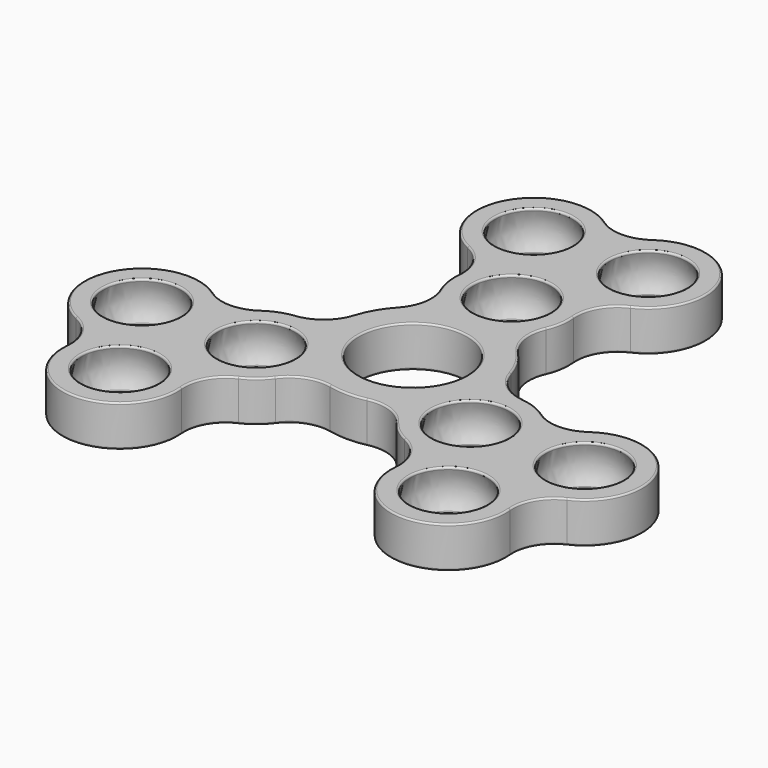
from build123d import *

# Parameters (mm, degrees)
F0_R     = 2.5
F0_R_2   = 6.56
F1_DEPTH = 2.5
F2_DEPTH = 2.5
F22_R    = 0.2


with BuildPart() as f1:
    # F0 (on Top) → F1 (new body)
    with BuildSketch(Plane.XY):
        with BuildLine():
            ThreePointArc((66.8263440398, 12.8050629308), (67.1732713624, 9.9684029043), (65.9098289008, 7.4050629308))
            ThreePointArc((65.9098289008, 7.4050629308), (64.5816959749, 5.6050629308), (63.686916711, 3.5548660774))
            ThreePointArc((63.686916711, 3.5548660774), (62.0987204063, 1.1790228227), (59.4686371001, 0.0611406841))
            ThreePointArc((59.4686371001, 0.0611406841), (57.7608978106, -0.3530293011), (56.2101170716, -1.1794610027))
            ThreePointArc((56.2101170716, -1.1794610027), (53.3233657257, -2.096978098), (50.4366143798, -1.1794610027))
            ThreePointArc((50.4366143798, -1.1794610027), (40.3329846689, -3.3949370692), (43.4661409693, -13.2526751024))
            ThreePointArc((43.4661409693, -13.2526751024), (45.7041097552, -15.2939165547), (46.3528923152, -18.2526751024))
            ThreePointArc((46.3528923152, -18.2526751024), (53.3233657257, -25.8949370692), (60.2938391362, -18.2526751024))
            ThreePointArc((60.2938391362, -18.2526751024), (60.9426216962, -15.2939165547), (63.1805904821, -13.2526751024))
            ThreePointArc((63.1805904821, -13.2526751024), (64.6716916996, -12.3228754376), (65.884243073, -11.0510148224))
            ThreePointArc((65.884243073, -11.0510148224), (68.1673990566, -9.3322369345), (71.019037823, -9.1447402157))
            ThreePointArc((71.019037823, -9.1447402157), (73.2419500127, -9.3949370692), (75.4648622025, -9.1447402157))
            ThreePointArc((75.4648622025, -9.1447402157), (78.3165009689, -9.3322369345), (80.5996569524, -11.0510148224))
            ThreePointArc((80.5996569524, -11.0510148224), (81.8122083259, -12.3228754376), (83.3033095434, -13.2526751024))
            ThreePointArc((83.3033095434, -13.2526751024), (85.5412783293, -15.2939165547), (86.1900608893, -18.2526751024))
            ThreePointArc((86.1900608893, -18.2526751024), (93.1605342998, -25.8949370692), (100.1310077103, -18.2526751024))
            ThreePointArc((100.1310077103, -18.2526751024), (100.7797902702, -15.2939165547), (103.0177590562, -13.2526751024))
            ThreePointArc((103.0177590562, -13.2526751024), (106.1509153566, -3.3949370692), (96.0472856457, -1.1794610027))
            ThreePointArc((96.0472856457, -1.1794610027), (93.1605342998, -2.096978098), (90.2737829538, -1.1794610027))
            ThreePointArc((90.2737829538, -1.1794610027), (88.7230022149, -0.3530293011), (87.0152629254, 0.0611406841))
            ThreePointArc((87.0152629254, 0.0611406841), (84.3851796192, 1.1790228227), (82.7969833144, 3.5548660774))
            ThreePointArc((82.7969833144, 3.5548660774), (81.9022040506, 5.6050629308), (80.5740711247, 7.4050629308))
            ThreePointArc((80.5740711247, 7.4050629308), (79.3106286631, 9.9684029043), (79.6575559857, 12.8050629308))
            ThreePointArc((79.6575559857, 12.8050629308), (80.1527439018, 14.4910935312), (80.2124234232, 16.2473248976))
            ThreePointArc((80.2124234232, 16.2473248976), (80.8612059832, 19.2060834453), (83.0991747692, 21.2473248976))
            ThreePointArc((83.0991747692, 21.2473248976), (86.2323310695, 31.1050629308), (76.1287013587, 33.3205389973))
            ThreePointArc((76.1287013587, 33.3205389973), (73.2419500127, 32.403021902), (70.3551986668, 33.3205389973))
            ThreePointArc((70.3551986668, 33.3205389973), (60.251568956, 31.1050629308), (63.3847252563, 21.2473248976))
            ThreePointArc((63.3847252563, 21.2473248976), (65.6226940423, 19.2060834453), (66.2714766023, 16.2473248976))
            ThreePointArc((66.2714766023, 16.2473248976), (66.3311561237, 14.4910935312), (66.8263440398, 12.8050629308))
        make_face()
        with Locations((53.3233657257, -18.8949370692)):
            Circle(F0_R, mode=Mode.SUBTRACT)
        with Locations((46.3951624954, -6.8949370692)):
            Circle(F0_R, mode=Mode.SUBTRACT)
        with Locations((60.251568956, -6.8949370692)):
            Circle(F0_R, mode=Mode.SUBTRACT)
        with Locations((73.2419500127, 0.6050629308)):
            Circle(F0_R_2, mode=Mode.SUBTRACT)
        with Locations((93.1605342998, -18.8949370692)):
            Circle(F0_R, mode=Mode.SUBTRACT)
        with Locations((86.2323310695, -6.8949370692)):
            Circle(F0_R, mode=Mode.SUBTRACT)
        with Locations((100.0887375301, -6.8949370692)):
            Circle(F0_R, mode=Mode.SUBTRACT)
        with Locations((73.2419500127, 15.6050629308)):
            Circle(F0_R, mode=Mode.SUBTRACT)
        with Locations((66.3137467825, 27.6050629308)):
            Circle(F0_R, mode=Mode.SUBTRACT)
        with Locations((80.170153243, 27.6050629308)):
            Circle(F0_R, mode=Mode.SUBTRACT)
    extrude(amount=F1_DEPTH)

    # F0 (on Top) → F2 (join)
    with BuildSketch(Plane.XY):
        with BuildLine():
            ThreePointArc((66.8263440398, 12.8050629308), (67.1732713624, 9.9684029043), (65.9098289008, 7.4050629308))
            ThreePointArc((65.9098289008, 7.4050629308), (64.5816959749, 5.6050629308), (63.686916711, 3.5548660774))
            ThreePointArc((63.686916711, 3.5548660774), (62.0987204063, 1.1790228227), (59.4686371001, 0.0611406841))
            ThreePointArc((59.4686371001, 0.0611406841), (57.7608978106, -0.3530293011), (56.2101170716, -1.1794610027))
            ThreePointArc((56.2101170716, -1.1794610027), (53.3233657257, -2.096978098), (50.4366143798, -1.1794610027))
            ThreePointArc((50.4366143798, -1.1794610027), (40.3329846689, -3.3949370692), (43.4661409693, -13.2526751024))
            ThreePointArc((43.4661409693, -13.2526751024), (45.7041097552, -15.2939165547), (46.3528923152, -18.2526751024))
            ThreePointArc((46.3528923152, -18.2526751024), (53.3233657257, -25.8949370692), (60.2938391362, -18.2526751024))
            ThreePointArc((60.2938391362, -18.2526751024), (60.9426216962, -15.2939165547), (63.1805904821, -13.2526751024))
            ThreePointArc((63.1805904821, -13.2526751024), (64.6716916996, -12.3228754376), (65.884243073, -11.0510148224))
            ThreePointArc((65.884243073, -11.0510148224), (68.1673990566, -9.3322369345), (71.019037823, -9.1447402157))
            ThreePointArc((71.019037823, -9.1447402157), (73.2419500127, -9.3949370692), (75.4648622025, -9.1447402157))
            ThreePointArc((75.4648622025, -9.1447402157), (78.3165009689, -9.3322369345), (80.5996569524, -11.0510148224))
            ThreePointArc((80.5996569524, -11.0510148224), (81.8122083259, -12.3228754376), (83.3033095434, -13.2526751024))
            ThreePointArc((83.3033095434, -13.2526751024), (85.5412783293, -15.2939165547), (86.1900608893, -18.2526751024))
            ThreePointArc((86.1900608893, -18.2526751024), (93.1605342998, -25.8949370692), (100.1310077103, -18.2526751024))
            ThreePointArc((100.1310077103, -18.2526751024), (100.7797902702, -15.2939165547), (103.0177590562, -13.2526751024))
            ThreePointArc((103.0177590562, -13.2526751024), (106.1509153566, -3.3949370692), (96.0472856457, -1.1794610027))
            ThreePointArc((96.0472856457, -1.1794610027), (93.1605342998, -2.096978098), (90.2737829538, -1.1794610027))
            ThreePointArc((90.2737829538, -1.1794610027), (88.7230022149, -0.3530293011), (87.0152629254, 0.0611406841))
            ThreePointArc((87.0152629254, 0.0611406841), (84.3851796192, 1.1790228227), (82.7969833144, 3.5548660774))
            ThreePointArc((82.7969833144, 3.5548660774), (81.9022040506, 5.6050629308), (80.5740711247, 7.4050629308))
            ThreePointArc((80.5740711247, 7.4050629308), (79.3106286631, 9.9684029043), (79.6575559857, 12.8050629308))
            ThreePointArc((79.6575559857, 12.8050629308), (80.1527439018, 14.4910935312), (80.2124234232, 16.2473248976))
            ThreePointArc((80.2124234232, 16.2473248976), (80.8612059832, 19.2060834453), (83.0991747692, 21.2473248976))
            ThreePointArc((83.0991747692, 21.2473248976), (86.2323310695, 31.1050629308), (76.1287013587, 33.3205389973))
            ThreePointArc((76.1287013587, 33.3205389973), (73.2419500127, 32.403021902), (70.3551986668, 33.3205389973))
            ThreePointArc((70.3551986668, 33.3205389973), (60.251568956, 31.1050629308), (63.3847252563, 21.2473248976))
            ThreePointArc((63.3847252563, 21.2473248976), (65.6226940423, 19.2060834453), (66.2714766023, 16.2473248976))
            ThreePointArc((66.2714766023, 16.2473248976), (66.3311561237, 14.4910935312), (66.8263440398, 12.8050629308))
        make_face()
        with Locations((53.3233657257, -18.8949370692)):
            Circle(F0_R, mode=Mode.SUBTRACT)
        with Locations((46.3951624954, -6.8949370692)):
            Circle(F0_R, mode=Mode.SUBTRACT)
        with Locations((60.251568956, -6.8949370692)):
            Circle(F0_R, mode=Mode.SUBTRACT)
        with Locations((73.2419500127, 0.6050629308)):
            Circle(F0_R_2, mode=Mode.SUBTRACT)
        with Locations((93.1605342998, -18.8949370692)):
            Circle(F0_R, mode=Mode.SUBTRACT)
        with Locations((86.2323310695, -6.8949370692)):
            Circle(F0_R, mode=Mode.SUBTRACT)
        with Locations((100.0887375301, -6.8949370692)):
            Circle(F0_R, mode=Mode.SUBTRACT)
        with Locations((73.2419500127, 15.6050629308)):
            Circle(F0_R, mode=Mode.SUBTRACT)
        with Locations((66.3137467825, 27.6050629308)):
            Circle(F0_R, mode=Mode.SUBTRACT)
        with Locations((80.170153243, 27.6050629308)):
            Circle(F0_R, mode=Mode.SUBTRACT)
    extrude(amount=-F2_DEPTH)


with BuildPart() as f4:
    # F3 (on face) → F4 (revolve)
    with BuildSketch(Plane.XY):
        with BuildLine():
            Line((53.3233657257, -24.1049370692), (53.3233657257, -18.8949370692))
            Line((53.3233657257, -18.8949370692), (53.3233657257, -13.6849370692))
            ThreePointArc((53.3233657257, -13.6849370692), (48.1133657257, -18.8949370692), (53.3233657257, -24.1049370692))
        make_face()
    revolve(axis=Axis((53.3233657257, -16.2899370692, 0), (0, 1, 0)))


with BuildPart() as f7:
    # F6 (on face) → F7 (revolve)
    with BuildSketch(Plane.XY):
        with BuildLine():
            Line((93.1605342998, -24.1049370692), (93.1605342998, -18.8949370692))
            Line((93.1605342998, -18.8949370692), (93.1605342998, -13.6849370692))
            ThreePointArc((93.1605342998, -13.6849370692), (87.9505342998, -18.8949370692), (93.1605342998, -24.1049370692))
        make_face()
    revolve(axis=Axis((93.1605342998, -16.2899370692, 0), (0, 1, 0)))


with BuildPart() as f9:
    # F8 (on face) → F9 (revolve)
    with BuildSketch(Plane.XY):
        with BuildLine():
            Line((86.2323310695, -12.1049370692), (86.2323310695, -6.8949370692))
            Line((86.2323310695, -6.8949370692), (86.2323310695, -1.6849370692))
            ThreePointArc((86.2323310695, -1.6849370692), (81.0223310695, -6.8949370692), (86.2323310695, -12.1049370692))
        make_face()
    revolve(axis=Axis((86.2323310695, -4.2899370692, 0), (0, 1, 0)))


with BuildPart() as f11:
    # F10 (on face) → F11 (revolve)
    with BuildSketch(Plane.XY):
        with BuildLine():
            Line((100.0887375301, -12.1049370692), (100.0887375301, -6.8949370692))
            Line((100.0887375301, -6.8949370692), (100.0887375301, -1.6849370692))
            ThreePointArc((100.0887375301, -1.6849370692), (94.8787375301, -6.8949370692), (100.0887375301, -12.1049370692))
        make_face()
    revolve(axis=Axis((100.0887375301, -9.4999370692, 0), (0, -1, 0)))


with BuildPart() as f13:
    # F12 (on face) → F13 (revolve)
    with BuildSketch(Plane.XY):
        with BuildLine():
            Line((73.2419500127, 10.3950629308), (73.2419500127, 15.6050629308))
            Line((73.2419500127, 15.6050629308), (73.2419500127, 20.8150629308))
            ThreePointArc((73.2419500127, 20.8150629308), (68.0319500127, 15.6050629308), (73.2419500127, 10.3950629308))
        make_face()
    revolve(axis=Axis((73.2419500127, 13.0000629308, 0), (0, -1, 0)))


with BuildPart() as f15:
    # F14 (on face) → F15 (revolve)
    with BuildSketch(Plane.XY):
        with BuildLine():
            Line((66.3137467825, 22.3950629308), (66.3137467825, 27.6050629308))
            Line((66.3137467825, 27.6050629308), (66.3137467825, 32.8150629308))
            ThreePointArc((66.3137467825, 32.8150629308), (61.1037467825, 27.6050629308), (66.3137467825, 22.3950629308))
        make_face()
    revolve(axis=Axis((66.3137467825, 25.0000629308, 0), (0, -1, 0)))


with BuildPart() as f17:
    # F5 (on face) → F17 (revolve)
    with BuildSketch(Plane.XY):
        with BuildLine():
            Line((60.251568956, -12.1049370692), (60.251568956, -6.8949370692))
            Line((60.251568956, -6.8949370692), (60.251568956, -1.6849370692))
            ThreePointArc((60.251568956, -1.6849370692), (55.041568956, -6.8949370692), (60.251568956, -12.1049370692))
        make_face()
    revolve(axis=Axis((60.251568956, -4.2899370692, 0), (0, 1, 0)))


with BuildPart() as f18:
    # F16 (on face) → F18 (revolve)
    with BuildSketch(Plane.XY):
        with BuildLine():
            Line((80.170153243, 22.3950629308), (80.170153243, 27.6050629308))
            Line((80.170153243, 27.6050629308), (80.170153243, 32.8150629308))
            ThreePointArc((80.170153243, 32.8150629308), (74.960153243, 27.6050629308), (80.170153243, 22.3950629308))
        make_face()
    revolve(axis=Axis((80.170153243, 25.0000629308, 0), (0, -1, 0)))


with BuildPart() as f20:
    # F19 (on face) → F20 (revolve)
    with BuildSketch(Plane.XY):
        with BuildLine():
            Line((46.3951624954, -12.1049370692), (46.3951624954, -6.8949370692))
            Line((46.3951624954, -6.8949370692), (46.3951624954, -1.6849370692))
            ThreePointArc((46.3951624954, -1.6849370692), (41.1851624954, -6.8949370692), (46.3951624954, -12.1049370692))
        make_face()
    revolve(axis=Axis((46.3951624954, -9.4999370692, 0), (0, -1, 0)))


with BuildPart() as f1_1:
    add(f1.part)

    # F21: cut F15, F18, F13, F9, F11, F20, F17, F4, F7
    add(f15.part, mode=Mode.SUBTRACT)
    add(f18.part, mode=Mode.SUBTRACT)
    add(f13.part, mode=Mode.SUBTRACT)
    add(f9.part, mode=Mode.SUBTRACT)
    add(f11.part, mode=Mode.SUBTRACT)
    add(f20.part, mode=Mode.SUBTRACT)
    add(f17.part, mode=Mode.SUBTRACT)
    add(f4.part, mode=Mode.SUBTRACT)
    add(f7.part, mode=Mode.SUBTRACT)

    # F22
    f22_edges = [f1_1.edges().sort_by_distance(p)[0] for p in [
        (60.251569, 31.105063, 2.5),
        (73.24195, 32.403022, 2.5),
        (65.622694, 19.206083, 2.5),
        (86.232331, 31.105063, 2.5),
        (66.331156, 14.491094, 2.5),
        (80.861206, 19.206083, 2.5),
        (67.173271, 9.968403, 2.5),
        (80.152744, 14.491094, 2.5),
        (64.581696, 5.605063, 2.5),
        (79.310629, 9.968403, 2.5),
        (62.09872, 1.179023, 2.5),
        (81.902204, 5.605063, 2.5),
        (57.760898, -0.353029, 2.5),
        (84.38518, 1.179023, 2.5),
        (53.323366, -2.096978, 2.5),
        (88.723002, -0.353029, 2.5),
        (40.332985, -3.394937, 2.5),
        (93.160534, -2.096978, 2.5),
        (45.70411, -15.293917, 2.5),
        (106.150915, -3.394937, 2.5),
        (53.323366, -25.894937, 2.5),
        (100.77979, -15.293917, 2.5),
        (60.942622, -15.293917, 2.5),
        (93.160534, -25.894937, 2.5),
        (64.671692, -12.322875, 2.5),
        (85.541278, -15.293917, 2.5),
        (68.167399, -9.332237, 2.5),
        (81.812208, -12.322875, 2.5),
        (73.24195, -9.394937, 2.5),
        (78.316501, -9.332237, 2.5),
        (53.323366, -14.323931, 2.5),
        (46.395162, -2.323931, 2.5),
        (60.251569, -2.323931, 2.5),
        (93.160534, -14.323931, 2.5),
        (86.232331, -2.323931, 2.5),
        (66.68195, 0.605063, 2.5),
        (100.088738, -2.323931, 2.5),
        (73.24195, 20.176069, 2.5),
        (66.313747, 32.176069, 2.5),
        (80.170153, 32.176069, 2.5),
        (60.251569, 31.105063, -2.5),
        (73.24195, 32.403022, -2.5),
        (65.622694, 19.206083, -2.5),
        (86.232331, 31.105063, -2.5),
        (66.331156, 14.491094, -2.5),
        (80.861206, 19.206083, -2.5),
        (67.173271, 9.968403, -2.5),
        (80.152744, 14.491094, -2.5),
        (64.581696, 5.605063, -2.5),
        (79.310629, 9.968403, -2.5),
        (62.09872, 1.179023, -2.5),
        (81.902204, 5.605063, -2.5),
        (57.760898, -0.353029, -2.5),
        (84.38518, 1.179023, -2.5),
        (53.323366, -2.096978, -2.5),
        (88.723002, -0.353029, -2.5),
        (40.332985, -3.394937, -2.5),
        (93.160534, -2.096978, -2.5),
        (45.70411, -15.293917, -2.5),
        (106.150915, -3.394937, -2.5),
        (53.323366, -25.894937, -2.5),
        (100.77979, -15.293917, -2.5),
        (60.942622, -15.293917, -2.5),
        (93.160534, -25.894937, -2.5),
        (64.671692, -12.322875, -2.5),
        (85.541278, -15.293917, -2.5),
        (68.167399, -9.332237, -2.5),
        (81.812208, -12.322875, -2.5),
        (73.24195, -9.394937, -2.5),
        (78.316501, -9.332237, -2.5),
        (53.323366, -14.323931, -2.5),
        (46.395162, -2.323931, -2.5),
        (60.251569, -2.323931, -2.5),
        (93.160534, -14.323931, -2.5),
        (86.232331, -2.323931, -2.5),
        (66.68195, 0.605063, -2.5),
        (100.088738, -2.323931, -2.5),
        (73.24195, 20.176069, -2.5),
        (66.313747, 32.176069, -2.5),
        (80.170153, 32.176069, -2.5),
    ]]
    fillet(f22_edges, radius=F22_R)


solid = f1_1.part
